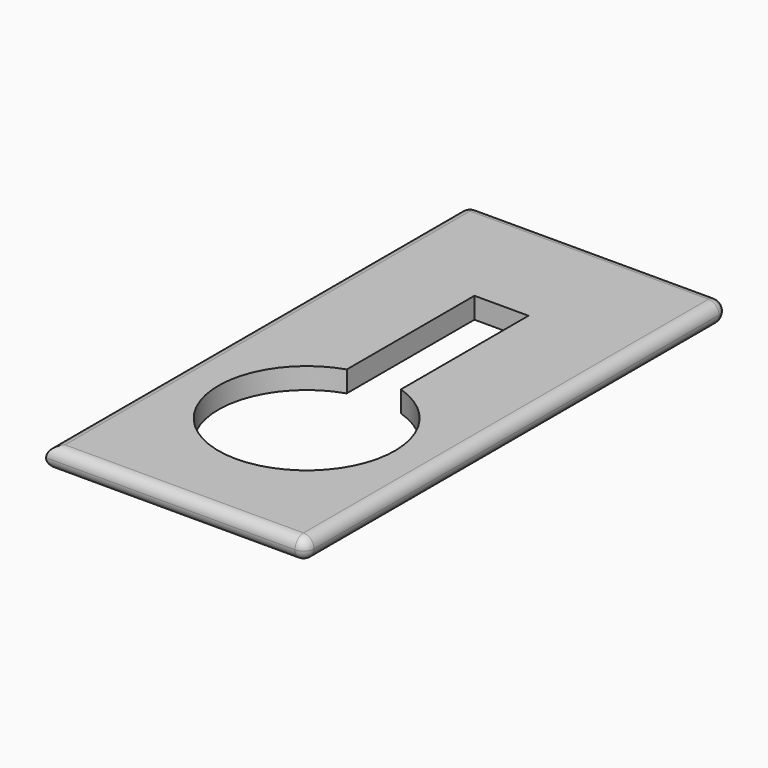
from build123d import *

# Parameters (mm, degrees)
F0_W     = 125
F0_H     = 254
F1_DEPTH = 10.16
F2_R     = 5.07999


# Not quite as in the source:
# - a fillet or chamfer is up to 0.001 mm smaller than in the source, because OpenCascade refuses the exact size


with BuildPart() as f1:
    # F0 (on Top) → F1 (new body)
    with BuildSketch(Plane.XY):
        with Locations((0, 7.7496204972)):
            Rectangle(F0_W, F0_H)
        with BuildLine():
            ThreePointArc((12.9974298287, 0), (34.3412344545, -15.4252090897), (42.5, -40.4637716711))
            ThreePointArc((42.5, -40.4637716711), (-25.0385625813, -74.8050061256), (-12.9974298287, 0))
            Line((-12.9974298287, 0), (-13.0543755367, 0))
            Line((-13.0543755367, 0), (-13.0543755367, 76.8597647548))
            Line((-13.0543755367, 76.8597647548), (12.9974298287, 76.8597647548))
            Line((12.9974298287, 76.8597647548), (12.9974298287, 0))
        make_face(mode=Mode.SUBTRACT)
    extrude(amount=F1_DEPTH)

    # F2 (radius 5.08 in the source; OpenCascade refuses exactly that, so slightly less here)
    f2_edges = [f1.edges().sort_by_distance(p)[0] for p in [
        (0, 134.74962, 10.16),
        (-62.5, 134.74962, 5.08),
        (-62.5, 7.74962, 10.16),
        (62.5, 7.74962, 10.16),
        (0, -119.25038, 10.16),
        (-62.5, 7.74962, 0),
        (62.5, -119.25038, 5.08),
        (62.5, 134.74962, 5.08),
        (62.5, 7.74962, 0),
        (0, -119.25038, 0),
        (0, 134.74962, 0),
    ]]
    fillet(f2_edges, radius=F2_R)


solid = f1.part
